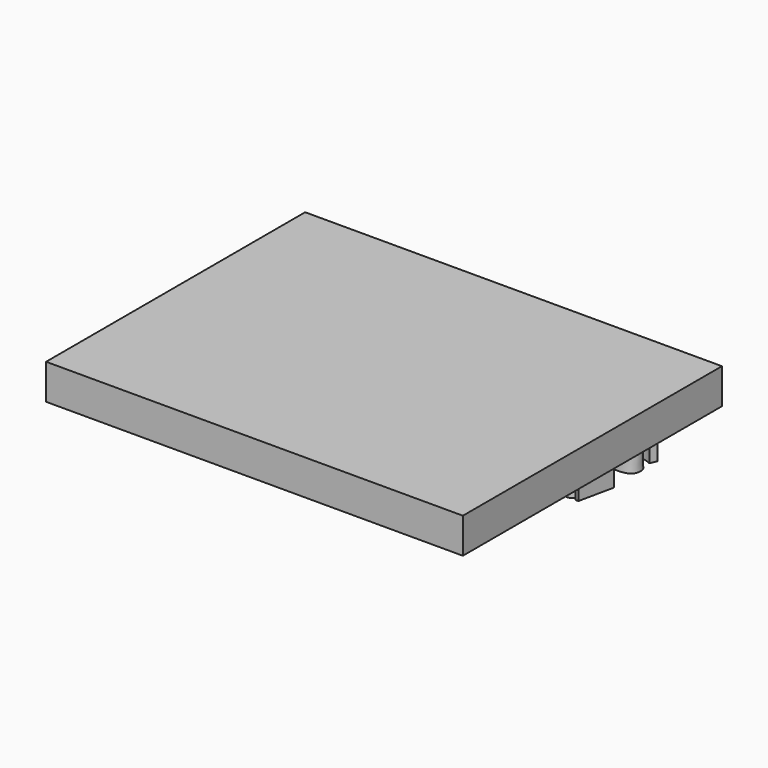
from build123d import *

# Parameters (mm, degrees)
F0_W         = 65
F0_H         = 50.5
F1_DEPTH     = 5.5
F2_TEXT_SIZE = 9.5142255969
F3_DEPTH     = 3
F4_TEXT_SIZE = 7.1931250324
F5_DEPTH     = 8.5


# Not quite as in the source:
# - Text() gives the source's letters only with a copy of the font that has no kerning and outlines rounded to 1/6400 em; it was checked with that copy


with BuildPart() as f1:
    # F0 (on Top) → F1 (new body)
    with BuildSketch(Plane.XY):
        Rectangle(F0_W, F0_H)
    extrude(amount=F1_DEPTH)

    # F2 (on Top) → F3 (join)
    with BuildSketch(Plane.XY):
        with Locations((-32.5, 8.6275720809)):
            Text('The Perlmans', F2_TEXT_SIZE, font='Open Sans', font_style=FontStyle.BOLD, text_align=(TextAlign.LEFT, TextAlign.BOTTOM))
    extrude(amount=-F3_DEPTH)

    # F4 (on face) → F5 (join)
    with BuildSketch(Plane.XY.offset(5.5)):
        with Locations((-32.5, -0.7007336612)):
            Text('1346 Stratford Road', F4_TEXT_SIZE, font='Open Sans', font_style=FontStyle.ITALIC, text_align=(TextAlign.LEFT, TextAlign.BOTTOM))
        with Locations((-30.6309114174, -10.4833837053)):
            Text('Deerfield, IL 60015', F4_TEXT_SIZE, font='Open Sans', font_style=FontStyle.ITALIC, text_align=(TextAlign.LEFT, TextAlign.BOTTOM))
    extrude(amount=-F5_DEPTH)


solid = f1.part
